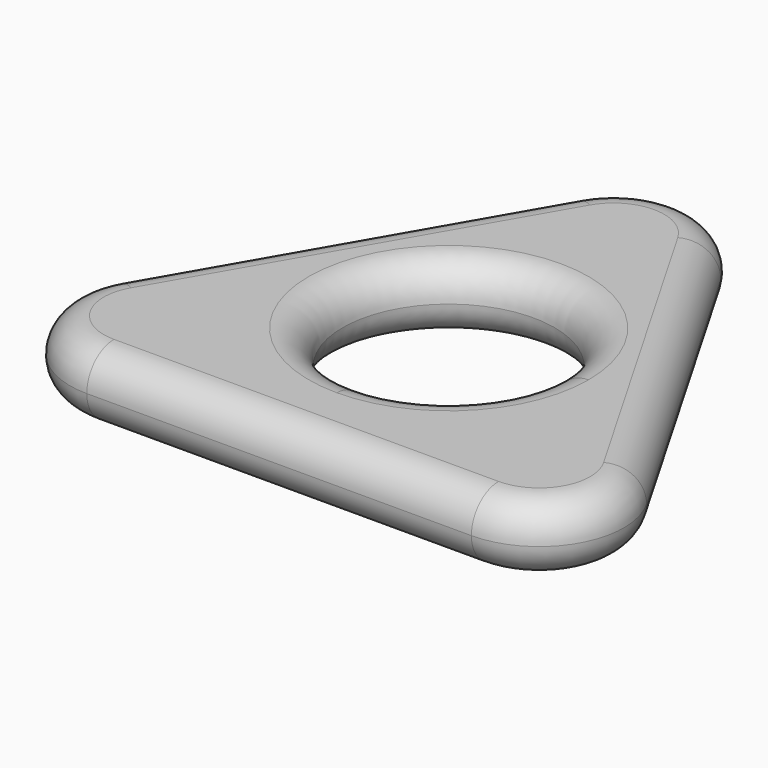
from build123d import *

# Parameters (mm, degrees)
F1_DEPTH = 4
F2_R     = 10
F3_R     = 3.99999


# Not quite as in the source:
# - a fillet or chamfer is up to 0.001 mm smaller than in the source, because OpenCascade refuses the exact size


with BuildPart() as f1:
    # F0 (on Top) → F1 (new body)
    with BuildSketch(Plane.XY):
        Polygon((40, -25), (0, 44.2820323028), (-40, -25), (0, -25), align=None)
        with BuildLine():
            ThreePointArc((12.5, 0), (8.8388347648, -8.8388347648), (0, -12.5))
            ThreePointArc((0, -12.5), (-8.8388347648, 8.8388347648), (12.5, 0))
        make_face(mode=Mode.SUBTRACT)
    extrude(amount=F1_DEPTH)

    # F2
    f2_edges = [f1.edges().sort_by_distance(p)[0] for p in [
        (0, 44.282032, 2),
        (-40, -25, 2),
        (40, -25, 2),
    ]]
    fillet(f2_edges, radius=F2_R)

    # F3 (radius 4 in the source; OpenCascade refuses exactly that, so slightly less here)
    f3_edges = [f1.edges().sort_by_distance(p)[0] for p in [
        (-12.5, 0, 4),
        (20, 9.641016, 4),
        (31.339746, -20, 4),
        (0, 34.282032, 4),
        (0, -25, 4),
        (-20, 9.641016, 4),
        (-31.339746, -20, 4),
    ]]
    fillet(f3_edges, radius=F3_R)


with BuildPart() as f4_1:
    # F4: instance of F1
    add(f1.part.mirror(Plane.XY))


solid = Compound([f1.part, f4_1.part])
